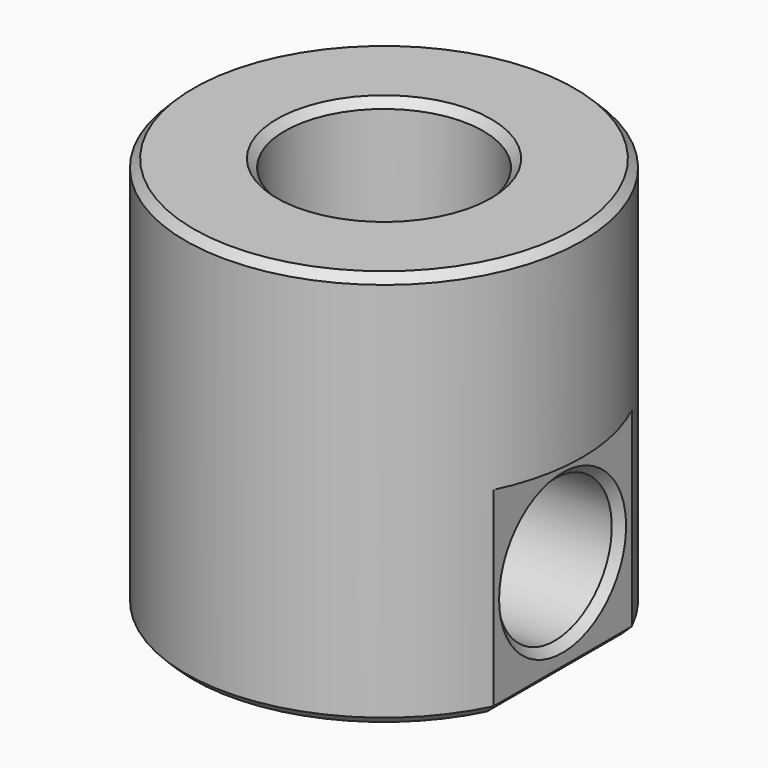
from build123d import *

# Parameters (mm, degrees)
F0_R     = 25
F1_DEPTH = 50
F2_W     = 23.745389397
F2_H     = 47.3247256844
F2_W_2   = 14.1143929356
F3_DEPTH = 25
F5_D     = 18
F6_R     = 12.5
F7_DEPTH = 25
F8_SIZE  = 1


with BuildPart() as f1:
    # F0 (on Top) → F1 (new body)
    with BuildSketch(Plane.XY):
        Circle(F0_R)
    extrude(amount=F1_DEPTH)

    # F2 (on Top) → F3 (cut)
    with BuildSketch(Plane.XY):
        with Locations((34.3726946985, 1.0396027938)):
            Rectangle(F2_W, F2_H)
        with Locations((-29.5571964678, 1.0396027938)):
            Rectangle(F2_W_2, F2_H)
    extrude(amount=F3_DEPTH, mode=Mode.SUBTRACT)

    # F5 (through all)
    with Locations(Plane.YZ.offset(22.5)):
        with Locations((0, 12.5)):
            Hole(F5_D / 2)

    # F6 (on face) → F7 (cut)
    with BuildSketch(Plane.XY.offset(50)):
        Circle(F6_R)
    extrude(amount=-F7_DEPTH, mode=Mode.SUBTRACT)

    # F8
    f8_edges = [f1.edges().sort_by_distance(p)[0] for p in [
        (-25, 0, 50),
        (0, 25, 0),
        (0, -25, 0),
        (22.5, 0, 0),
        (-22.5, 0, 0),
        (-12.5, 0, 50),
        (22.5, -9, 12.5),
        (-22.5, -9, 12.5),
    ]]
    chamfer(f8_edges, length=F8_SIZE)


solid = f1.part
